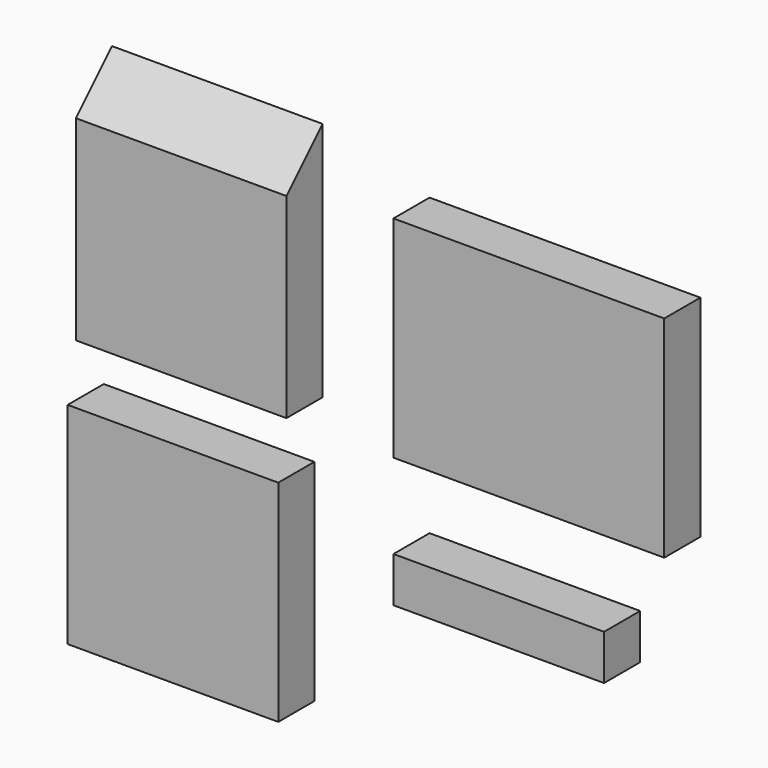
from build123d import *

# Parameters (mm, degrees)
F0_W     = 114.3
F0_H     = 88.9
F1_DEPTH = 19.05
F2_W     = 88.9
F2_H     = 19.05
F3_DEPTH = 19.05
F4_W     = 88.9
F4_H     = 101.6
F5_DEPTH = 19.05
F7_DEPTH = 248.3578988337
F8_W     = 88.9
F8_H     = 88.9
F9_DEPTH = 19.05


with BuildPart() as f1:
    # F0 (on Front) → F1 (new body)
    with BuildSketch(Plane.XZ):
        with Locations((57.15, 44.45)):
            Rectangle(F0_W, F0_H)
    extrude(amount=F1_DEPTH)


with BuildPart() as f3:
    # F2 (on Front) → F3 (new body)
    with BuildSketch(Plane.XZ):
        with Locations((44.45, -45.3105017608)):
            Rectangle(F2_W, F2_H)
    extrude(amount=F3_DEPTH)


with BuildPart() as f5:
    # F4 (on Front) → F5 (new body)
    with BuildSketch(Plane.XZ):
        with Locations((-89.6068988337, 50.8)):
            Rectangle(F4_W, F4_H)
    extrude(amount=F5_DEPTH)

    # F6 (on face) → F7 (cut, through all)
    with BuildSketch(Plane(origin=(-134.0568988337, 0, 0), x_dir=(0, -1, 0), z_dir=(-1, 0, 0))):
        Polygon((19.05, 101.6), (0, 101.6), (19.05, 82.55), align=None)
    extrude(amount=-F7_DEPTH, mode=Mode.SUBTRACT)


with BuildPart() as f9:
    # F8 (on Front) → F9 (new body)
    with BuildSketch(Plane.XZ):
        with Locations((-93.0538623974, -69.5413928479)):
            Rectangle(F8_W, F8_H)
    extrude(amount=F9_DEPTH)


solid = Compound([f1.part, f3.part, f5.part, f9.part])
